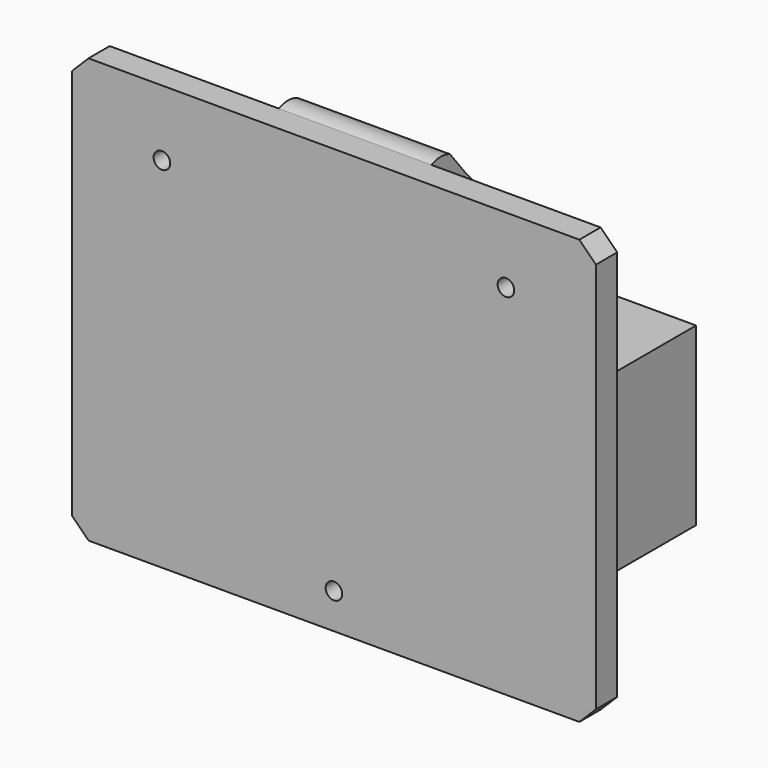
from build123d import *

# Parameters (mm, degrees)
F0_W     = 116
F0_H     = 53
F1_DEPTH = 52
F3_DEPTH = 23
F4_R     = 2.5
F5_DEPTH = 8
F6_SIZE  = 5
F7_W     = 46
F7_H     = 12.914198093
F8_DEPTH = 4


# Not quite as in the source:
# - a feature names something its author has since deleted; it is built from what else it names


with BuildPart() as f1:
    # F0 (on Front) → F1 (new body)
    with BuildSketch(Plane.XZ):
        with Locations((0, 8.5)):
            Rectangle(F0_W, F0_H)
    extrude(amount=F1_DEPTH)

    # F2 (on Right) → F3 (join, symmetric)
    with BuildSketch(Plane.YZ):
        with BuildLine():
            Line((-45, 35), (0, 35))
            Line((0, 35), (0, 47.914198093))
            ThreePointArc((0, 47.914198093), (-24.3783358313, 66.3998162753), (-45, 89))
            Line((-45, 89), (-45, 35))
        make_face()
        with BuildLine():
            Line((-52, 35), (-45, 35))
            Line((-45, 35), (-45, 89))
            ThreePointArc((-45, 89), (-48.5, 89.7722433198), (-52, 89))
            Line((-52, 89), (-52, 35))
        make_face()
    extrude(amount=F3_DEPTH, both=True)

    # F4 (on face) → F5 (join)
    with BuildSketch(Plane.XZ.offset(52)):
        Polygon((-23, 89), (-79, 89), (-79, -39), (79, -39), (79, 89), (23, 89), (23, 35), (58, 35), (58, -18), (-58, -18), (-58, 35), (-23, 35), align=None)
        with Locations((0, -28.3078663051)):
            Circle(F4_R, mode=Mode.SUBTRACT)
        with Locations((-51.8612675369, 69.1157281399)):
            Circle(F4_R, mode=Mode.SUBTRACT)
        with Locations((51.8612675369, 69.1157281399)):
            Circle(F4_R, mode=Mode.SUBTRACT)
        Polygon((23, 89), (-23, 89), (-23, 35), (-58, 35), (-58, -18), (58, -18), (58, 35), (23, 35), align=None)
    extrude(amount=F5_DEPTH)

    # F6
    f6_edges = [f1.edges().sort_by_distance(p)[0] for p in [
        (-79, -56, 89),
        (79, -56, 89),
        (79, -56, -39),
        (-79, -56, -39),
    ]]
    chamfer(f6_edges, length=F6_SIZE)

    # F7 (on face) → F8 (join)
    with BuildSketch(Plane(origin=(0, 0, 0), x_dir=(-1, 0, 0), z_dir=(0, 1, 0))):
        with Locations((0, 41.4570990465)):
            Rectangle(F7_W, F7_H)
        Polygon((-23, 35), (-58, 35), (-58, -18), (58, -18), (58, 35), (23, 35), align=None)
    extrude(amount=F8_DEPTH)


solid = f1.part
